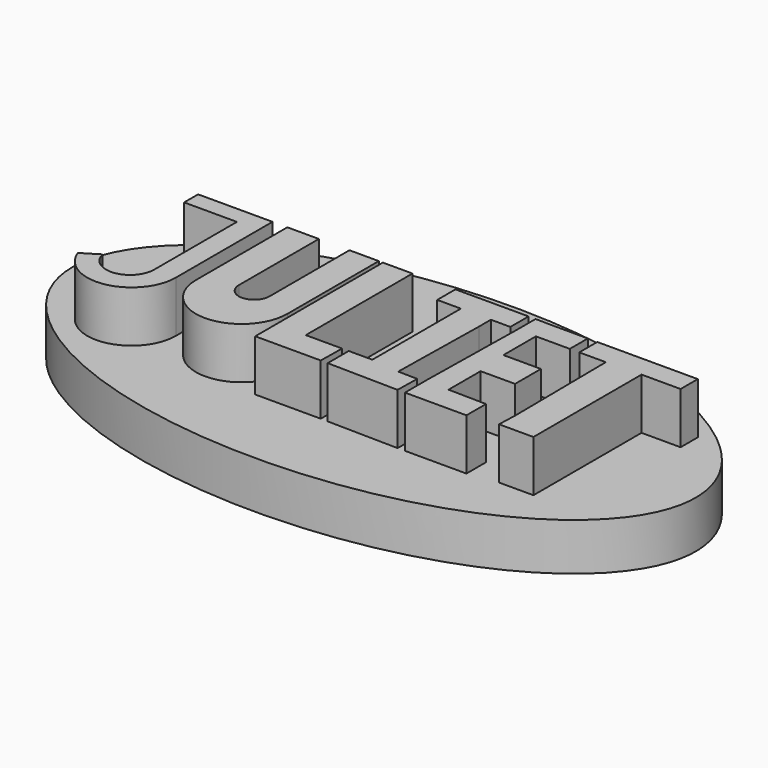
from build123d import *

# Parameters (mm, degrees)
F1_DEPTH = 25
F3_DEPTH = 12
F4_SCALE = 1.25
F6_D     = 5


with BuildPart() as f1:
    # F0 (on Top) → F1 (new body)
    with BuildSketch(Plane.XY):
        with BuildLine():
            Line((-13.2980933413, 65.3656870127), (-20.7502059639, 65.3656870127))
            Line((-20.7502059639, 65.3656870127), (-20.7502059639, 40.0356650352))
            ThreePointArc((-20.7502059639, 40.0356650352), (-24.6234871447, 36.1623838544), (-28.4967683256, 40.0356650352))
            Line((-28.4967683256, 40.0356650352), (-28.4967683256, 65.3656870127))
            Line((-28.4967683256, 65.3656870127), (-31.6937640309, 65.3656870127))
            Line((-31.6937640309, 65.3656870127), (-36.4933647215, 65.3656870127))
            Line((-36.4933647215, 65.3656870127), (-36.4933647215, 36.3845080137))
            ThreePointArc((-36.4933647215, 36.3845080137), (-24.8957290314, 24.7868723236), (-13.2980933413, 36.3845080137))
            Line((-13.2980933413, 36.3845080137), (-13.2980933413, 65.3656870127))
        make_face()
    extrude(amount=F1_DEPTH)



with BuildPart() as f1b:
    # F0 (on Top) → F1, piece 2 (new body)
    with BuildSketch(Plane.XY):
        Polygon((-4.7652381472, 65.3656870127), (-12.2658768669, 65.3656870127), (-12.2658768669, 30.3217209876), (-12.2658768669, 24.9114241451), (4.3338974938, 24.9114241451), (4.4483790145, 31.551335007), (-4.7652381472, 31.551335007), (-4.7652381472, 37.9453226924), (-4.7652381472, 61.2577274442), align=None)
    extrude(amount=F1_DEPTH)


with BuildPart() as f1c:
    # F0 (on Top) → F1, piece 3 (new body)
    with BuildSketch(Plane.XY):
        Polygon((67.6116645336, 65.3051072577), (42.1355515718, 65.3051072577), (42.1355515718, 59.5998801291), (48.8598830998, 59.5998801291), (49.1652822897, 30.7737427528), (48.9826314151, 25.598635897), (57.7109195292, 25.598635897), (57.7109195292, 59.8604232073), (67.6116645336, 59.8604232073), align=None)
    extrude(amount=F1_DEPTH)


with BuildPart() as f1d:
    # F0 (on Top) → F1, piece 4 (new body)
    with BuildSketch(Plane.XY):
        Polygon((29.9600720621, 65.3051072577), (26.4464554486, 65.3656870127), (26.4464554486, 59.5998801291), (25.9677926885, 31.8375125559), (25.9677926885, 30.6562086032), (25.9677926885, 25.2078175545), (25.9677926885, 24.5709556187), (41.5497215959, 24.5709556187), (41.5497215959, 24.9391629061), (41.5497215959, 30.7737427528), (31.9168753922, 30.9398267418), (31.9168753922, 41.1011204123), (40.6451635063, 41.1011204123), (40.6451635063, 49.3083149195), (31.1352387071, 49.3083149195), (31.1352387071, 59.5998801291), (39.7332534194, 59.5998801291), (39.7332534194, 64.1594305634), (39.7332534194, 65.3051072577), align=None)
    extrude(amount=F1_DEPTH)


with BuildPart() as f1e:
    # F0 (on Top) → F1, piece 5 (new body)
    with BuildSketch(Plane.XY):
        Polygon((24.081020448, 24.5709556187), (24.1864684053, 30.6869211711), (19.2915876022, 30.7713158881), (19.7249674405, 55.9072808625), (19.7249674405, 59.5998801291), (24.6661454439, 59.5998801291), (24.6661454439, 65.3656870127), (12.5062046573, 65.3656870127), (6.1232019216, 65.3656870127), (6.1232019216, 59.5998801291), (12.115384452, 59.5998801291), (12.115384452, 55.4311461747), (12.115384452, 31.551335007), (6.4647817053, 31.551335007), (6.1232019216, 31.551335007), (6.1232019216, 24.8805739882), align=None)
    extrude(amount=F1_DEPTH)


with BuildPart() as f1f:
    # F0 (on Top) → F1, piece 6 (new body)
    with BuildSketch(Plane.XY):
        with BuildLine():
            Line((-40.2501347491, 38.9378666878), (-40.2501347491, 65.3656870127))
            Line((-40.2501347491, 65.3656870127), (-59.1141320765, 65.3656870127))
            Line((-59.1141320765, 65.3656870127), (-59.1141320765, 60.9390847385))
            Line((-59.1141320765, 60.9390847385), (-45.7351878285, 60.9390847385))
            Line((-45.7351878285, 60.9390847385), (-45.7351878285, 40.1110313833))
            Line((-45.7351878285, 40.1110313833), (-45.7351878285, 37.0055958629))
            Line((-45.7351878285, 37.0055958629), (-45.7351878285, 34.7282737494))
            ThreePointArc((-45.7351878285, 34.7282737494), (-51.1972258986, 28.6670752331), (-57.7922141434, 33.471044153))
            Line((-57.7922141434, 33.471044153), (-62.0269551873, 30.8637320995))
            ThreePointArc((-62.0269551873, 30.8637320995), (-49.5189871635, 23.6697409515), (-40.2501347491, 34.7282737494))
            Line((-40.2501347491, 34.7282737494), (-40.2501347491, 37.0055958629))
            Line((-40.2501347491, 37.0055958629), (-40.2501347491, 38.9378666878))
        make_face()
    extrude(amount=F1_DEPTH)


with BuildPart() as f1_1:
    add(f1.part)

    add(f1b.part)  # F3 merges F1b

    add(f1c.part)  # F3 merges F1c

    add(f1d.part)  # F3 merges F1d

    add(f1e.part)  # F3 merges F1e

    add(f1f.part)  # F3 merges F1f
    # F2 (on Top) → F3 (join)
    with BuildSketch(Plane.XY):
        with BuildLine():
            add(Edge.make_bspline(
                [(-74.6536329389, 44.8788292706), (-74.6536329389, -26.5993963968), (43.9336113632, 9.1397164369), (162.5208556652, 44.8788292706), (43.9336113632, 80.6179421043), (-74.6536329389, 116.357054938), (-74.6536329389, 44.8788292706)],
                knots=[0, 0, 0, 2.0943951024, 2.0943951024, 4.1887902048, 4.1887902048, 6.2831853072, 6.2831853072, 6.2831853072], degree=2, weights=[1, 0.5, 1, 0.5, 1, 0.5, 1]))
        make_face()
    extrude(amount=F3_DEPTH)


with BuildPart() as f1_2:
    # F4: moved
    add(f1_1.part.scale(F4_SCALE).moved(Location((-1.5308004804, -16.3414217532, 0))))

    # F6 (through all)
    with Locations(Plane(origin=(0, 0, 0), x_dir=(1, 0, 0), z_dir=(0, 0, -1))):
        with Locations((-36.0251380689, -75.7874920964), (3.9748619311, -75.7874920964), (43.9748619311, -75.7874920964)):
            Hole(F6_D / 2)


solid = f1_2.part
